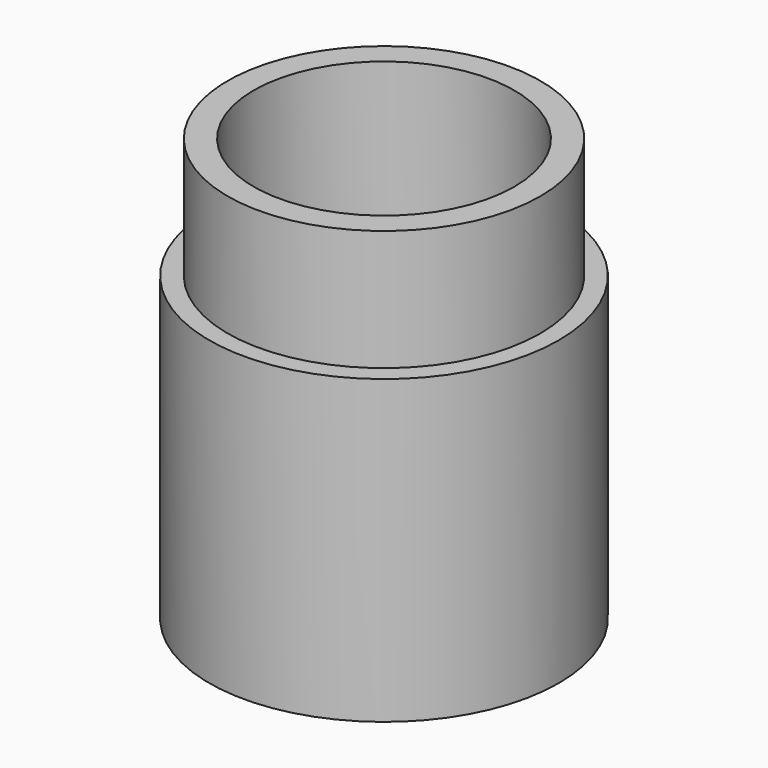
from build123d import *

# Parameters (mm, degrees)
F0_R          = 14.48
F1_DEPTH      = 25
F2_R          = 12.5
F3_DEPTH      = 22
F4_R          = 9
F5_DEPTH      = 3
F6_R          = 12.5
F7_DEPTH      = 1
F8_R          = 12.95
F9_DEPTH      = 10
F10_R         = 10.8
F11_DEPTH     = 11
F12_S5_R      = 10.8
F12_T6_DEPTH  = 19
F12_S11_R     = 9
F12_T12_DEPTH = 19


# Not quite as in the source:
# - a fillet or chamfer that OpenCascade refuses, or shapes differently, is made with other operations: its cross-section is extruded or revolved along the edge and cut away or added


with BuildPart() as f1:
    # F0 (on Top) → F1 (new body)
    with BuildSketch(Plane.XY):
        Circle(F0_R)
    extrude(amount=F1_DEPTH)

    # F2 (on face) → F3 (cut)
    with BuildSketch(Plane.XY.offset(25)):
        Circle(F2_R)
    extrude(amount=-F3_DEPTH, mode=Mode.SUBTRACT)

    # F4 (on face) → F5 (cut, through all)
    with BuildSketch(Plane(origin=(0, 0, 0), x_dir=(1, 0, 0), z_dir=(0, 0, -1))):
        Circle(F4_R)
    extrude(amount=-F5_DEPTH, mode=Mode.SUBTRACT)

    # F6 (on face) → F7 (join)
    with BuildSketch(Plane.XY.offset(25)):
        Circle(F6_R)
    extrude(amount=-F7_DEPTH)

    # F8 (on face) → F9 (join)
    with BuildSketch(Plane.XY.offset(25)):
        Circle(F8_R)
    extrude(amount=F9_DEPTH)

    # F10 (on face) → F11 (cut, through all)
    with BuildSketch(Plane.XY.offset(35)):
        Circle(F10_R)
    extrude(amount=-F11_DEPTH, mode=Mode.SUBTRACT)

    # F12: chamfer of 5 on 3 edges, made by hand


with BuildPart() as f12_tool2:
    # F12_s3 → F12_t4 (revolve)
    with BuildSketch(Plane.XZ):
        Polygon((12.5, 19), (7.5, 24), (12.5, 24), align=None)
    revolve(axis=Axis((0, 0, 24), (0, 0, 1)))

    # F12_s5 → F12_t6 (cut, symmetric)
    with BuildSketch(Plane.XY.offset(21.5)):
        Circle(F12_S5_R)
    extrude(amount=F12_T6_DEPTH, both=True, mode=Mode.SUBTRACT)


with BuildPart() as f1_1:
    add(f1.part)

    # F12_t1: union F12_tool2
    add(f12_tool2.part)


with BuildPart() as f12_tool8:
    # F12_s9 → F12_t10 (revolve)
    with BuildSketch(Plane.XZ):
        Polygon((7.5, 3), (12.5, 8), (12.5, 3), align=None)
    revolve(axis=Axis((0, 0, 3), (0, 0, 1)))

    # F12_s11 → F12_t12 (cut, symmetric)
    with BuildSketch(Plane.XY.offset(5.5)):
        Circle(F12_S11_R)
    extrude(amount=F12_T12_DEPTH, both=True, mode=Mode.SUBTRACT)


with BuildPart() as f1_2:
    add(f1_1.part)

    # F12_t7: union F12_tool8
    add(f12_tool8.part)


solid = f1_2.part
